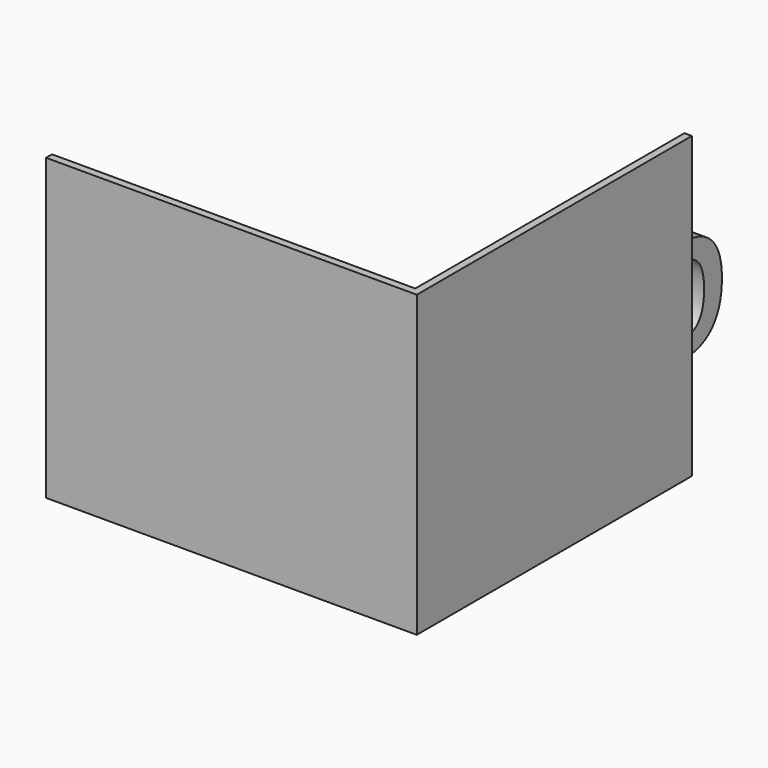
from build123d import *

# Parameters (mm, degrees)
F1_DEPTH     = 101.6
F2_T         = -2.54
F3_TEXT_SIZE = 47.6350283457
F4_DEPTH     = 25.4


# Not quite as in the source:
# - Text() gives the source's letters only with a copy of the font that has no kerning and outlines rounded to 1/6400 em; it was checked with that copy


with BuildPart() as f1:
    # F0 (on Top) → F1 (new body)
    with BuildSketch(Plane.XY):
        with BuildLine():
            ThreePointArc((0, 0), (-43.2889174701, 17.9308567165), (-61.2197741866, 61.2197741866))
            Line((-61.2197741866, 61.2197741866), (-61.2197741866, -55.4614774883))
            Line((-61.2197741866, -55.4614774883), (64.5535215735, -55.4614774883))
            Line((64.5535215735, -55.4614774883), (64.5535215735, 61.2197741866))
            ThreePointArc((64.5535215735, 61.2197741866), (20.0703284018, 43.4810256554), (0, 0))
        make_face()
        with BuildLine():
            Line((64.5535215735, 61.2197741866), (-61.2197741866, 61.2197741866))
            ThreePointArc((-61.2197741866, 61.2197741866), (-43.2889174701, 17.9308567165), (0, 0))
            ThreePointArc((0, 0), (20.0703284018, 43.4810256554), (64.5535215735, 61.2197741866))
        make_face()
    extrude(amount=F1_DEPTH)

    # F2
    f2_openings = [f1.faces().sort_by_distance(p)[0] for p in [
        (1.666874, 2.879148, 0),
        (-61.219774, 2.879148, 50.8),
        (1.666874, 61.219774, 50.8),
        (1.666874, 2.879148, 101.6),
    ]]
    offset(amount=F2_T, openings=f2_openings)

    # F3 (on face) → F4 (join)
    with BuildSketch(Plane(origin=(62.0135215735, 0, 0), x_dir=(0, -1, 0), z_dir=(-1, 0, 0))):
        with Locations((-79.9090005457, 34.6219353378)):
            Text('Open', F3_TEXT_SIZE, font='Open Sans', font_style=FontStyle.BOLD, text_align=(TextAlign.LEFT, TextAlign.BOTTOM))
    extrude(amount=F4_DEPTH)


solid = f1.part
